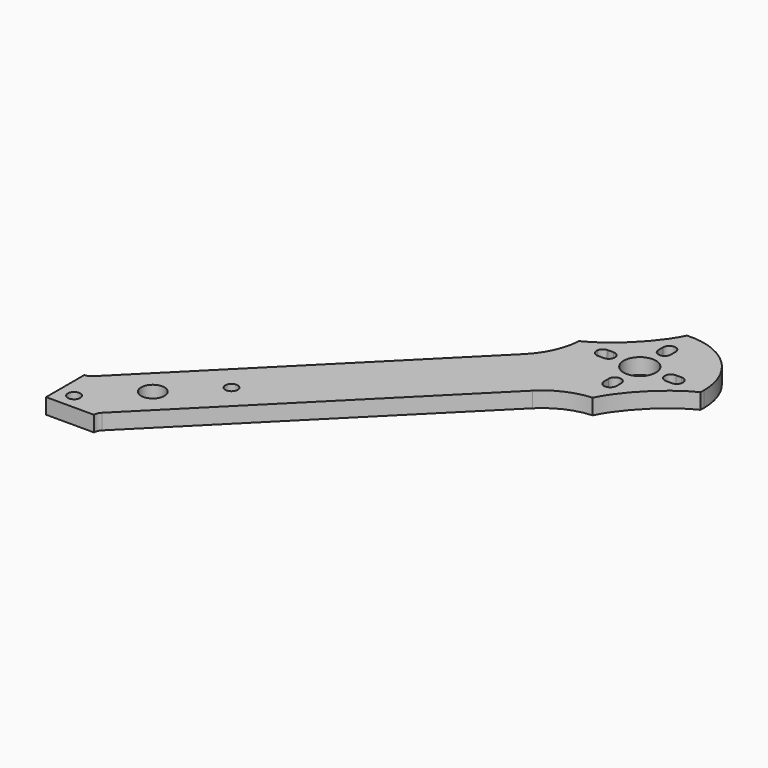
from build123d import *

# Parameters (mm, degrees)
F0_R        = 1.6
F0_R_2      = 3
F1_DEPTH    = 4
F2_T1_DEPTH = 4
F3_R        = 2.4


# Not quite as in the source:
# - a fillet or chamfer that OpenCascade refuses, or shapes differently, is made with other operations: its cross-section is extruded or revolved along the edge and cut away or added


with BuildPart() as f1:
    # F0 (on Top) → F1 (new body)
    with BuildSketch(Plane.XY):
        with BuildLine():
            ThreePointArc((80.3055021759, 68.9917936769), (73.1855518528, 73.1855518528), (68.9917936769, 80.3055021759))
            Line((68.9917936769, 80.3055021759), (1, 12.313708499))
            Line((1, 12.313708499), (0, 11.313708499))
            Line((0, 11.313708499), (0, 0))
            Line((0, 0), (11.313708499, 0))
            Line((11.313708499, 0), (12.313708499, 1))
            Line((12.313708499, 1), (80.3055021759, 68.9917936769))
        make_face()
        with Locations((4, 4)):
            Circle(F0_R, mode=Mode.SUBTRACT)
        with Locations((15.25, 15.25)):
            Circle(F0_R_2, mode=Mode.SUBTRACT)
        with Locations((26.499998178, 26.499998178)):
            Circle(F0_R, mode=Mode.SUBTRACT)
        with BuildLine():
            ThreePointArc((87.7873068843, 81.9183206005), (81.9183206005, 81.9183206005), (81.9183206005, 87.7873068843))
            Line((81.9183206005, 87.7873068843), (79.1959594929, 90.5096679919))
            Line((79.1959594929, 90.5096679919), (75.1224322345, 86.4361407335))
            ThreePointArc((75.1224322345, 86.4361407335), (75.2373217206, 86.4486400465), (75.3528137424, 86.4528137424))
            Line((75.3528137424, 86.4528137424), (76.8528137424, 86.4528137424))
            ThreePointArc((76.8528137424, 86.4528137424), (77.9841845923, 85.9841845923), (78.4528137424, 84.8528137424))
            ThreePointArc((78.4528137424, 84.8528137424), (77.9841845923, 83.7214428925), (76.8528137424, 83.2528137424))
            Line((76.8528137424, 83.2528137424), (75.3528137424, 83.2528137424))
            ThreePointArc((75.3528137424, 83.2528137424), (74.1427289494, 83.8060593329), (73.7694867513, 85.0831952502))
            Line((73.7694867513, 85.0831952502), (68.9917936769, 80.3055021759))
            ThreePointArc((68.9917936769, 80.3055021759), (73.1855518528, 73.1855518528), (80.3055021759, 68.9917936769))
            Line((80.3055021759, 68.9917936769), (85.0831952502, 73.7694867513))
            ThreePointArc((85.0831952502, 73.7694867513), (83.8060593329, 74.1427289494), (83.2528137424, 75.3528137424))
            Line((83.2528137424, 75.3528137424), (83.2528137424, 76.8528137424))
            ThreePointArc((83.2528137424, 76.8528137424), (84.8528137424, 78.4528137424), (86.4528137424, 76.8528137424))
            Line((86.4528137424, 76.8528137424), (86.4528137424, 75.3528137424))
            ThreePointArc((86.4528137424, 75.3528137424), (86.4486400465, 75.2373217206), (86.4361407335, 75.1224322345))
            Line((86.4361407335, 75.1224322345), (90.5096679919, 79.1959594929))
            Line((90.5096679919, 79.1959594929), (87.7873068843, 81.9183206005))
        make_face()
        with BuildLine():
            Line((79.1959594929, 90.5096679919), (81.9183206005, 87.7873068843))
            ThreePointArc((81.9183206005, 87.7873068843), (86.4409499867, 88.6869138023), (89.0028137424, 84.8528137424))
            ThreePointArc((89.0028137424, 84.8528137424), (88.6869138023, 83.2646774981), (87.7873068843, 81.9183206005))
            Line((87.7873068843, 81.9183206005), (90.5096679919, 79.1959594929))
            Line((90.5096679919, 79.1959594929), (86.4361407335, 75.1224322345))
            ThreePointArc((86.4361407335, 75.1224322345), (85.9841845923, 74.2214428925), (85.0831952502, 73.7694867513))
            Line((85.0831952502, 73.7694867513), (80.3055021759, 68.9917936769))
            ThreePointArc((80.3055021759, 68.9917936769), (83.083856654, 68.4479123157), (85.9142893623, 68.3869924902))
            add(Edge.make_bspline(
                [(101.3186349946, 83.7913381225), (90.8947856118, 78.810841873), (85.9142893623, 68.3869924902)],
                knots=[3.9431649716, 3.9431649716, 3.9431649716, 5.4816129892, 5.4816129892, 5.4816129892], degree=2, weights=[1, 0.7184506482, 1]))
            ThreePointArc((101.3186349946, 83.7913381225), (101.3442668418, 84.321800871), (101.3528137424, 84.8528137424))
            ThreePointArc((101.3528137424, 84.8528137424), (96.1385492583, 96.8895148629), (83.7913381225, 101.3186349946))
            add(Edge.make_bspline(
                [(68.3869924902, 85.9142893623), (78.810841873, 90.8947856118), (83.7913381225, 101.3186349946)],
                knots=[0.801572318, 0.801572318, 0.801572318, 2.3400203356, 2.3400203356, 2.3400203356], degree=2, weights=[1, 0.7184506482, 1]))
            ThreePointArc((68.3869924902, 85.9142893623), (68.4479123157, 83.083856654), (68.9917936769, 80.3055021759))
            Line((68.9917936769, 80.3055021759), (73.7694867513, 85.0831952502))
            ThreePointArc((73.7694867513, 85.0831952502), (74.2214428925, 85.9841845923), (75.1224322345, 86.4361407335))
            Line((75.1224322345, 86.4361407335), (79.1959594929, 90.5096679919))
        make_face()
        with BuildLine():
            ThreePointArc((95.9528137424, 84.8528137424), (95.4841845923, 83.7214428925), (94.3528137424, 83.2528137424))
            Line((94.3528137424, 83.2528137424), (92.8528137424, 83.2528137424))
            ThreePointArc((92.8528137424, 83.2528137424), (91.2528137424, 84.8528137424), (92.8528137424, 86.4528137424))
            Line((92.8528137424, 86.4528137424), (94.3528137424, 86.4528137424))
            ThreePointArc((94.3528137424, 86.4528137424), (95.4841845923, 85.9841845923), (95.9528137424, 84.8528137424))
        make_face(mode=Mode.SUBTRACT)
        with BuildLine():
            Line((83.2528137424, 92.8528137424), (83.2528137424, 94.3528137424))
            ThreePointArc((83.2528137424, 94.3528137424), (84.8528137424, 95.9528137424), (86.4528137424, 94.3528137424))
            Line((86.4528137424, 94.3528137424), (86.4528137424, 92.8528137424))
            ThreePointArc((86.4528137424, 92.8528137424), (84.8528137424, 91.2528137424), (83.2528137424, 92.8528137424))
        make_face(mode=Mode.SUBTRACT)
        Polygon((12.313708499, 0), (12.313708499, 1), (11.313708499, 0), align=None)
        Polygon((0, 11.313708499), (1, 12.313708499), (0, 12.313708499), align=None)
    extrude(amount=F1_DEPTH)

    # F2: fillet of radius 17.7 on 2 edges, made by hand

    # F2_s2 → F2_t1 (join)
    with BuildSketch(Plane.XY):
        with BuildLine():
            ThreePointArc((74.55426567, 63.240557171), (79.7659943294, 66.8474433344), (85.9142893623, 68.3869924902))
            ThreePointArc((85.9142893623, 68.3869924902), (83.083856654, 68.4479123157), (80.3055021759, 68.9917936769))
            Line((80.3055021759, 68.9917936769), (74.55426567, 63.240557171))
        make_face()
        with BuildLine():
            ThreePointArc((68.3869924902, 85.9142893623), (66.8474433344, 79.7659943294), (63.240557171, 74.55426567))
            Line((63.240557171, 74.55426567), (68.9917936769, 80.3055021759))
            ThreePointArc((68.9917936769, 80.3055021759), (68.4479123157, 83.083856654), (68.3869924902, 85.9142893623))
        make_face()
    extrude(amount=F2_T1_DEPTH)

    # F3
    f3_edges = [f1.edges().sort_by_distance(p)[0] for p in [
        (12.313708, 1, 2),
        (1, 12.313708, 2),
    ]]
    fillet(f3_edges, radius=F3_R)


solid = f1.part
